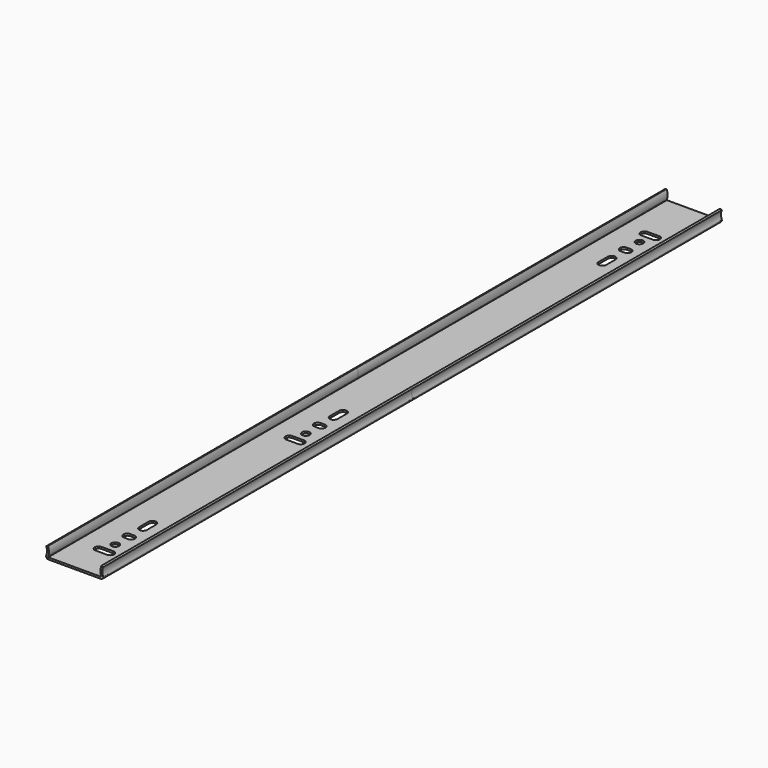
from build123d import *

# Parameters (mm, degrees)
F1_DEPTH     = 200
F2_R         = 2
F3_DEPTH     = 12.0270402445
F5_TEXT_SIZE = 9.5547634303
F6_DEPTH     = 0.4


# Not quite as in the source:
# - Text() gives the source's letters only with a copy of the font that has no kerning and outlines rounded to 1/6400 em; it was checked with that copy


with BuildPart() as f1:
    # F0 (on Front) → F1 (new body, symmetric)
    with BuildSketch(Plane.XZ):
        with BuildLine():
            add(Edge.make_bspline(
                [(-14.727593219, 11.6439480436), (-14.2682743707, 10.5330439332), (-14.1053562336, 8.6536075494), (-14.7859986702, 7.1970379958)],
                knots=[0, 0, 0, 0, 4.4472935781, 4.4472935781, 4.4472935781, 4.4472935781], degree=3))
            ThreePointArc((-14.7859986702, 7.1970379958), (-14.4685808768, 6.3131087443), (-13.6067331403, 5.939874962))
            Line((-13.6067331403, 5.939874962), (13.6067331403, 5.939874962))
            ThreePointArc((13.6067331403, 5.939874962), (14.4685808768, 6.3131087443), (14.7859986702, 7.1970379958))
            add(Edge.make_bspline(
                [(14.727593219, 11.6439480436), (14.2682743707, 10.5330439332), (14.1053562336, 8.6536075494), (14.7859986702, 7.1970379958)],
                knots=[0, 0, 0, 0, 4.4472935781, 4.4472935781, 4.4472935781, 4.4472935781], degree=3))
            Line((14.727593219, 11.6439480436), (13.8034689706, 12.0260401445))
            add(Edge.make_bspline(
                [(13.8034689706, 12.0260401445), (13.6585727295, 11.6755955012), (13.4335982949, 10.9042270809), (13.2887487964, 9.5814295855), (13.3817624549, 8.2597491442), (13.6168683346, 7.4066185146), (13.7664824472, 7.0350792406)],
                knots=[0, 0, 0, 0, 0.25, 0.5, 0.75, 0.9522436655, 0.9522436655, 0.9522436655, 0.9522436655], degree=3))
            ThreePointArc((13.7664824472, 7.0350792406), (13.6996987886, 6.965469543), (13.6066950322, 6.9398596163))
            Line((13.6066950322, 6.9398596163), (-13.6066950322, 6.9398596163))
            ThreePointArc((-13.6066950322, 6.9398596163), (-13.6996987886, 6.965469543), (-13.7664824472, 7.0350792406))
            add(Edge.make_bspline(
                [(-13.8034689706, 12.0260401445), (-13.6585727295, 11.6755955012), (-13.4335982949, 10.9042270809), (-13.2887487964, 9.5814295855), (-13.3817624549, 8.2597491442), (-13.6168683346, 7.4066185146), (-13.7664824472, 7.0350792406)],
                knots=[0, 0, 0, 0, 0.25, 0.5, 0.75, 0.9522436655, 0.9522436655, 0.9522436655, 0.9522436655], degree=3))
            Line((-13.8034689706, 12.0260401445), (-14.727593219, 11.6439480436))
        make_face()
    extrude(amount=F1_DEPTH, both=True)

    # F2 (on Top) → F3 (cut, through all)
    with BuildSketch(Plane.XY):
        with BuildLine():
            Line((-2.9814595297, -59.5609534753), (3.0185404703, -59.5609534753))
            ThreePointArc((3.0185404703, -59.5609534753), (4.4327540327, -58.9751670377), (5.0185404703, -57.5609534753))
            ThreePointArc((5.0185404703, -57.5609534753), (4.4327540327, -56.1467399129), (3.0185404703, -55.5609534753))
            Line((3.0185404703, -55.5609534753), (-2.9814595297, -55.5609534753))
            ThreePointArc((-2.9814595297, -55.5609534753), (-4.3956730921, -56.1467399129), (-4.9814595297, -57.5609534753))
            ThreePointArc((-4.9814595297, -57.5609534753), (-4.3956730921, -58.9751670377), (-2.9814595297, -59.5609534753))
        make_face()
        with Locations((0.0185404703, -50.5609534753)):
            Circle(F2_R)
        with BuildLine():
            Line((-1.0210410935, -43.5609534753), (0.9789589065, -43.5609534753))
            ThreePointArc((0.9789589065, -43.5609534753), (2.3931724688, -42.9751670377), (2.9789589065, -41.5609534753))
            ThreePointArc((2.9789589065, -41.5609534753), (2.3931724688, -40.1467399129), (0.9789589065, -39.5609534753))
            Line((0.9789589065, -39.5609534753), (-1.0210410935, -39.5609534753))
            ThreePointArc((-1.0210410935, -39.5609534753), (-2.4352546559, -40.1467399129), (-3.0210410935, -41.5609534753))
            ThreePointArc((-3.0210410935, -41.5609534753), (-2.4352546559, -42.9751670377), (-1.0210410935, -43.5609534753))
        make_face()
        with BuildLine():
            ThreePointArc((0.0185404703, -34.5609534753), (1.4327540327, -33.9751670377), (2.0185404703, -32.5609534753))
            Line((2.0185404703, -32.5609534753), (2.0185404703, -26.5609534753))
            ThreePointArc((2.0185404703, -26.5609534753), (1.4327540327, -25.1467399129), (0.0185404703, -24.5609534753))
            ThreePointArc((0.0185404703, -24.5609534753), (-1.3956730921, -25.1467399129), (-1.9814595297, -26.5609534753))
            Line((-1.9814595297, -26.5609534753), (-1.9814595297, -32.5609534753))
            ThreePointArc((-1.9814595297, -32.5609534753), (-1.3956730921, -33.9751670377), (0.0185404703, -34.5609534753))
        make_face()
        with BuildLine():
            ThreePointArc((0.521315504, -158.4240968585), (1.9355290664, -157.8383104209), (2.521315504, -156.4240968585))
            Line((2.521315504, -156.4240968585), (2.521315504, -150.4240968585))
            ThreePointArc((2.521315504, -150.4240968585), (1.9355290664, -149.0098832961), (0.521315504, -148.4240968585))
            ThreePointArc((0.521315504, -148.4240968585), (-0.8928980583, -149.0098832961), (-1.478684496, -150.4240968585))
            Line((-1.478684496, -150.4240968585), (-1.478684496, -156.4240968585))
            ThreePointArc((-1.478684496, -156.4240968585), (-0.8928980583, -157.8383104209), (0.521315504, -158.4240968585))
        make_face()
        with BuildLine():
            Line((-0.478684496, -167.4240968585), (1.521315504, -167.4240968585))
            ThreePointArc((1.521315504, -167.4240968585), (2.9355290664, -166.8383104209), (3.521315504, -165.4240968585))
            ThreePointArc((3.521315504, -165.4240968585), (2.9355290664, -164.0098832961), (1.521315504, -163.4240968585))
            Line((1.521315504, -163.4240968585), (-0.478684496, -163.4240968585))
            ThreePointArc((-0.478684496, -163.4240968585), (-1.8928980583, -164.0098832961), (-2.478684496, -165.4240968585))
            ThreePointArc((-2.478684496, -165.4240968585), (-1.8928980583, -166.8383104209), (-0.478684496, -167.4240968585))
        make_face()
        with BuildLine():
            ThreePointArc((0.521315504, -172.4240968585), (-0.8928980583, -173.0098832961), (-1.478684496, -174.4240968585))
            ThreePointArc((-1.478684496, -174.4240968585), (-0.8928980583, -175.8383104209), (0.521315504, -176.4240968585))
            ThreePointArc((0.521315504, -176.4240968585), (1.9355290664, -175.8383104209), (2.521315504, -174.4240968585))
            ThreePointArc((2.521315504, -174.4240968585), (1.9355290664, -173.0098832961), (0.521315504, -172.4240968585))
        make_face()
        with BuildLine():
            Line((-2.478684496, -183.4240968585), (3.521315504, -183.4240968585))
            ThreePointArc((3.521315504, -183.4240968585), (4.9355290664, -182.8383104209), (5.521315504, -181.4240968585))
            ThreePointArc((5.521315504, -181.4240968585), (4.9355290664, -180.0098832961), (3.521315504, -179.4240968585))
            Line((3.521315504, -179.4240968585), (-2.478684496, -179.4240968585))
            ThreePointArc((-2.478684496, -179.4240968585), (-3.8928980583, -180.0098832961), (-4.478684496, -181.4240968585))
            ThreePointArc((-4.478684496, -181.4240968585), (-3.8928980583, -182.8383104209), (-2.478684496, -183.4240968585))
        make_face()
        with BuildLine():
            ThreePointArc((0.5513158038, 148.4960092651), (-0.8628977585, 147.9102228275), (-1.4486841962, 146.4960092651))
            Line((-1.4486841962, 146.4960092651), (-1.4486841962, 140.4960092651))
            ThreePointArc((-1.4486841962, 140.4960092651), (-0.8628977585, 139.0817957027), (0.5513158038, 138.4960092651))
            ThreePointArc((0.5513158038, 138.4960092651), (1.9655293662, 139.0817957027), (2.5513158038, 140.4960092651))
            Line((2.5513158038, 140.4960092651), (2.5513158038, 146.4960092651))
            ThreePointArc((2.5513158038, 146.4960092651), (1.9655293662, 147.9102228275), (0.5513158038, 148.4960092651))
        make_face()
        with BuildLine():
            Line((1.5908973677, 157.4960092651), (-0.4091026323, 157.4960092651))
            ThreePointArc((-0.4091026323, 157.4960092651), (-1.8233161947, 156.9102228275), (-2.4091026323, 155.4960092651))
            ThreePointArc((-2.4091026323, 155.4960092651), (-1.8233161947, 154.0817957027), (-0.4091026323, 153.4960092651))
            Line((-0.4091026323, 153.4960092651), (1.5908973677, 153.4960092651))
            ThreePointArc((1.5908973677, 153.4960092651), (3.00511093, 154.0817957027), (3.5908973677, 155.4960092651))
            ThreePointArc((3.5908973677, 155.4960092651), (3.00511093, 156.9102228275), (1.5908973677, 157.4960092651))
        make_face()
        with Locations((0.5513158038, 164.4960092651)):
            Circle(F2_R)
        with BuildLine():
            Line((3.5513158038, 173.4960092651), (-2.4486841962, 173.4960092651))
            ThreePointArc((-2.4486841962, 173.4960092651), (-3.8628977585, 172.9102228275), (-4.4486841962, 171.4960092651))
            ThreePointArc((-4.4486841962, 171.4960092651), (-3.8628977585, 170.0817957027), (-2.4486841962, 169.4960092651))
            Line((-2.4486841962, 169.4960092651), (3.5513158038, 169.4960092651))
            ThreePointArc((3.5513158038, 169.4960092651), (4.9655293662, 170.0817957027), (5.5513158038, 171.4960092651))
            ThreePointArc((5.5513158038, 171.4960092651), (4.9655293662, 172.9102228275), (3.5513158038, 173.4960092651))
        make_face()
    extrude(amount=F3_DEPTH, mode=Mode.SUBTRACT)

    # F5 (on face) → F6 (cut)
    with BuildSketch(Plane(origin=(0, 0, 5.939874962), x_dir=(1, 0, 0), z_dir=(0, 0, -1))):
        with Locations(Location((-10.1179857512, -16.9479604078), (0, 0, -90))):
            Text('Slides this way -->', F5_TEXT_SIZE, font='Open Sans', text_align=(TextAlign.LEFT, TextAlign.BOTTOM))
    extrude(amount=-F6_DEPTH, mode=Mode.SUBTRACT)


solid = f1.part
